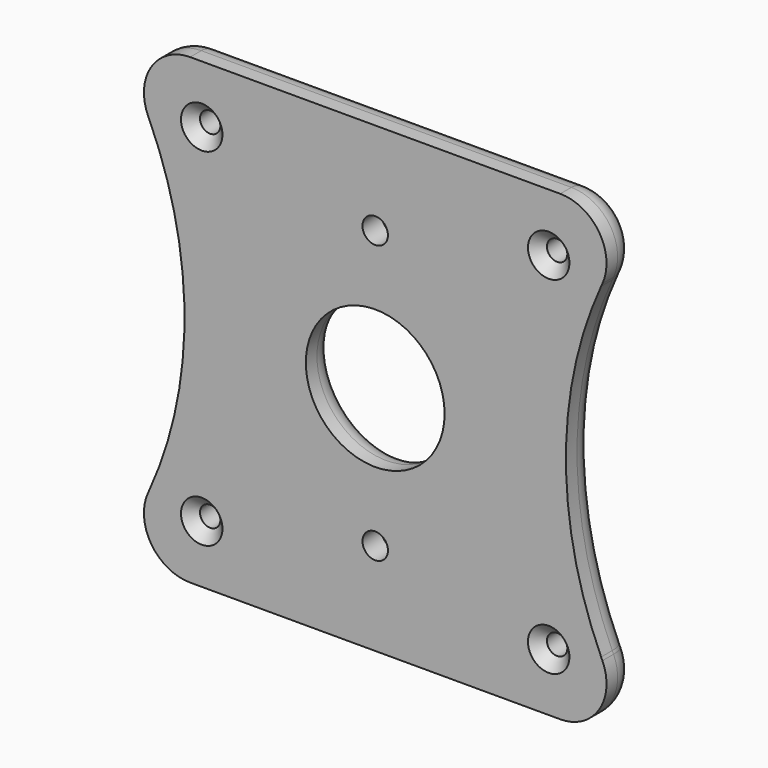
from build123d import *

# Parameters (mm, degrees)
F0_R           = 15
F1_DEPTH       = 8
F3_D           = 4.4
F3_START       = 2
F3_CSINK_D     = 8.96
F3_CSINK_ANGLE = 90
F5_D           = 5.5
F5_CSINK_D     = 11.2
F5_CSINK_ANGLE = 90
F6_R           = 5


# Not quite as in the source:
# - a feature names something its author has since deleted; it is built from what else it names


with BuildPart() as f1:
    # F0 (on Front) → F1 (new body)
    with BuildSketch(Plane.XZ):
        with BuildLine():
            Line((40, 50), (-40, 50))
            ThreePointArc((-40, 50), (-48.4035993498, 45.4202876277), (-49.1099851169, 35.8759035935))
            Line((-49.1099851169, 35.8759035935), (-48.8354949074, 35.2695642948))
            ThreePointArc((-48.8354949074, 35.2695642948), (-41.2240246484, 0), (-48.8354949074, -35.2695642948))
            Line((-48.8354949074, -35.2695642948), (-49.1099851169, -35.8759035935))
            ThreePointArc((-49.1099851169, -35.8759035935), (-48.4035993498, -45.4202876277), (-40, -50))
            Line((-40, -50), (40, -50))
            ThreePointArc((40, -50), (48.4035993498, -45.4202876277), (49.1099851169, -35.8759035935))
            Line((49.1099851169, -35.8759035935), (48.8354949074, -35.2695642948))
            ThreePointArc((48.8354949074, -35.2695642948), (41.2240246484, 0), (48.8354949074, 35.2695642948))
            Line((48.8354949074, 35.2695642948), (49.1099851169, 35.8759035935))
            ThreePointArc((49.1099851169, 35.8759035935), (48.4035993498, 45.4202876277), (40, 50))
        make_face()
        Circle(F0_R, mode=Mode.SUBTRACT)
    extrude(amount=F1_DEPTH)

    # F3 (through all)
    # its depths count from where the whole tool has entered the part; down to there all is cleared
    with Locations(Plane.XZ.offset(10).offset(-F3_START)):
        with Locations((-37.5, 37.5), (37.5, 37.5), (37.5, -37.5), (-37.5, -37.5)):
            CounterSinkHole(F3_D / 2, F3_CSINK_D / 2, counter_sink_angle=F3_CSINK_ANGLE)

    # F5 (through all)
    with Locations(Plane(origin=(0, 0, 0), x_dir=(-1, 0, 0), z_dir=(0, 1, 0))):
        with Locations((0, -30), (0, 30)):
            CounterSinkHole(F5_D / 2, F5_CSINK_D / 2, counter_sink_angle=F5_CSINK_ANGLE)

    # F6
    f6_edges = [f1.edges().sort_by_distance(p)[0] for p in [
        (0, 0, 50),
        (-15, 0, 0),
    ]]
    fillet(f6_edges, radius=F6_R)


solid = f1.part
